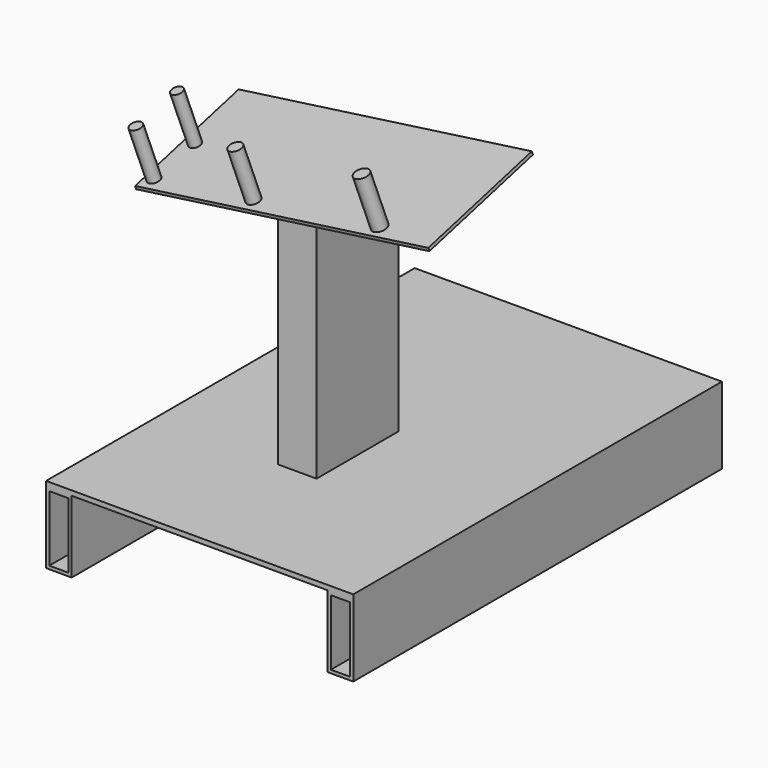
from build123d import *

# Parameters (mm, degrees)
F0_W      = 609.6
F0_H      = 914.4
F1_DEPTH  = 152.4
F2_W      = 508
F2_H      = 142.875
F3_DEPTH  = 914.401
F4_W      = 76.2
F4_H      = 203.2
F5_DEPTH  = 508
F7_DEPTH  = 322.6759463469
F8_SIZE2  = 76.19999
F8_SIZE   = 12.69999
F9_W      = 609.6
F9_H      = 264.8433126191
F10_DEPTH = 6.35
F11_R     = 12.0984700112
F11_R_2   = 11.4258541902
F11_R_3   = 13.0475001639
F11_R_4   = 14.3473050844
F12_DEPTH = 101.6
F13_DEPTH = 25.4
F14_W     = 38.1
F14_H     = 130.175
F15_DEPTH = 914.401


# Not quite as in the source:
# - a fillet or chamfer is up to 0.001 mm smaller than in the source, because OpenCascade refuses the exact size


with BuildPart() as f1:
    # F0 (on Top) → F1 (new body)
    with BuildSketch(Plane.XY):
        with Locations((20.2250536531, 87.9569677773)):
            Rectangle(F0_W, F0_H)
    extrude(amount=-F1_DEPTH)

    # F2 (on face) → F3 (cut, through all)
    with BuildSketch(Plane.XZ.offset(369.2430322227)):
        with Locations((20.2250536531, -80.9625)):
            Rectangle(F2_W, F2_H)
    extrude(amount=-F3_DEPTH, mode=Mode.SUBTRACT)

    # F4 (on face) → F5 (join)
    with BuildSketch(Plane.XY):
        Rectangle(F4_W, F4_H)
    extrude(amount=F5_DEPTH)

    # F6 (on face) → F7 (cut, through all)
    with BuildSketch(Plane.YZ.offset(38.1)):
        Polygon((-101.6, 469.9), (50.8, 508), (-101.6, 508), align=None)
    extrude(amount=-F7_DEPTH, mode=Mode.SUBTRACT)

    # F8 (size 12.7 and 76.2 in the source; OpenCascade refuses exactly that, so slightly less here)
    f8_edges = [f1.edges().sort_by_distance(p)[0] for p in [
        (-38.1, -25.4, 488.95),
    ]]
    chamfer(f8_edges, length=F8_SIZE, length2=F8_SIZE2)

    # F9 (on face) → F10 (join)
    with BuildSketch(Plane(origin=(-76.8910670792, -111.8929380826, 447.5717523306), x_dir=(0.9863939238, -0.0398726111, 0.1594904446), z_dir=(-0.1643989873, -0.2392356668, 0.9569426674))):
        with Locations((78.4772256914, 108.3081216617)):
            Rectangle(F9_W, F9_H)
    extrude(amount=F10_DEPTH)

    # F11 (on face) → F12 (join)
    with BuildSketch(Plane(origin=(-77.9350006486, -113.4120845671, 453.6483382685), x_dir=(0.9863939238, -0.0398726111, 0.1594904446), z_dir=(-0.1643989873, -0.2392356668, 0.9569426674))):
        with Locations((-206.5722942352, 0)):
            Circle(F11_R)
        with Locations((-200.9941935539, 98.414324224)):
            Circle(F11_R_2)
        with Locations((0, 0.4072751035)):
            Circle(F11_R_3)
        with Locations((262.7131342888, 0)):
            Circle(F11_R_4)
    extrude(amount=F12_DEPTH)

    # F11 (on face) → F13 (join)
    with BuildSketch(Plane(origin=(-77.9350006486, -113.4120845671, 453.6483382685), x_dir=(0.9863939238, -0.0398726111, 0.1594904446), z_dir=(-0.1643989873, -0.2392356668, 0.9569426674))):
        with Locations((-206.5722942352, 0)):
            Circle(F11_R)
        with Locations((-200.9941935539, 98.414324224)):
            Circle(F11_R_2)
        with Locations((0, 0.4072751035)):
            Circle(F11_R_3)
        with Locations((262.7131342888, 0)):
            Circle(F11_R_4)
    extrude(amount=F13_DEPTH)

    # F14 (on face) → F15 (cut, through all)
    with BuildSketch(Plane.XZ.offset(369.2430322227)):
        with Locations((-259.1749463469, -80.9625)):
            Rectangle(F14_W, F14_H)
        with Locations((299.6250536531, -80.9625)):
            Rectangle(F14_W, F14_H)
    extrude(amount=-F15_DEPTH, mode=Mode.SUBTRACT)


solid = f1.part
